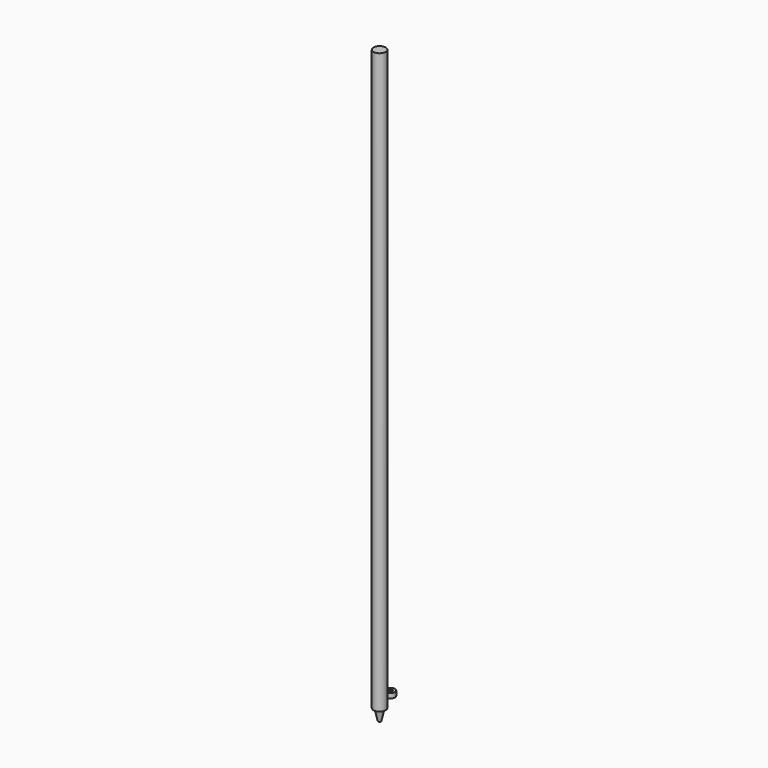
from build123d import *

# Parameters (mm, degrees)
F0_R     = 23
F0_R_2   = 10
F1_DEPTH = 25


# Not quite as in the source:
# - a feature names something its author has since deleted; it is built from what else it names


with BuildPart() as f1:
    # F0 (on Top) → F1 (new body)
    with BuildSketch(Plane.XY):
        Circle(F0_R)
        Circle(F0_R_2, mode=Mode.SUBTRACT)
    extrude(amount=F1_DEPTH)


with BuildPart() as f3:
    # F2 (on Right) → F3 (revolve)
    with BuildSketch(Plane.YZ):
        Polygon((-72.7435579151, 3013.7323013039), (-104.7435579151, 3013.7323013039), (-104.7435579151, -26.2676986961), (-94.361692667, -26.2676986961), (-80.2435579151, -86.7242515087), (-72.7435579151, -86.7242515087), (-72.7435579151, -63.013613224), (-72.7435579151, -26.2676986961), align=None)
    revolve(axis=Axis((0, -72.7435579151, 1493.7323013039), (0, 0, -1)))


solid = Compound([f1.part, f3.part])
